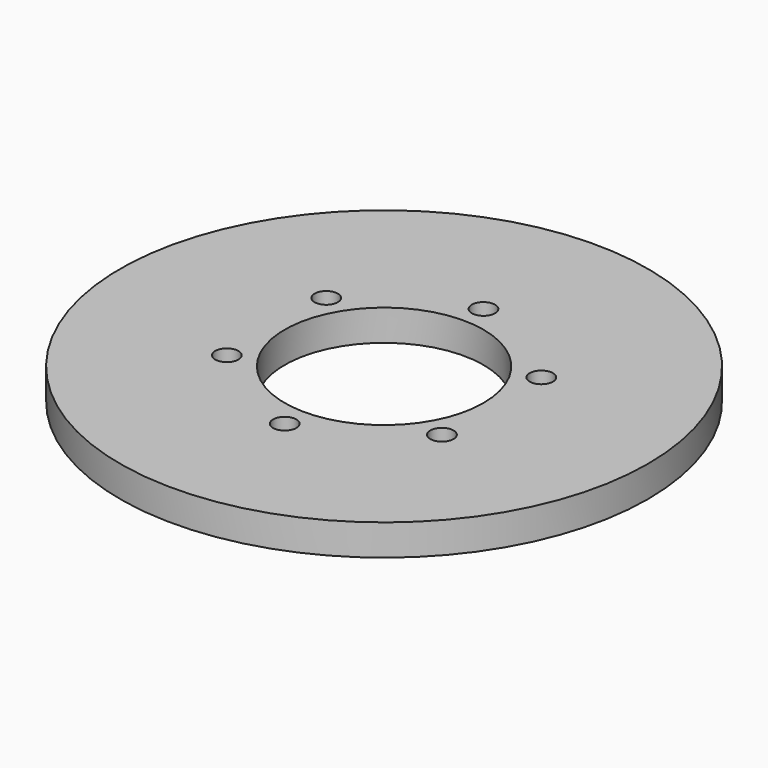
from build123d import *

# Parameters (mm, degrees)
F0_R            = 53.975
F0_R_2          = 20.32
F1_DEPTH        = 6.35
F2_D            = 4.7625
F2_DEPTH        = 6.35
F2_TIP          = 1.4307993491
F2_COPIES_COUNT = 6


# Not quite as in the source:
# - a pattern or mirror of a feature is missing from the dataset's text; its kind, count and spacing are read off the source's solid


with BuildPart() as f1:
    # F0 (on Top) → F1 (new body)
    with BuildSketch(Plane.XY):
        Circle(F0_R)
        Circle(F0_R_2, mode=Mode.SUBTRACT)
    extrude(amount=F1_DEPTH)

    # F2
    with Locations(Plane(origin=(0, 0, 0), x_dir=(1, 0, 0), z_dir=(0, 0, -1))):
        with Locations((0, 25.4)):
            f2 = Hole(F2_D / 2, depth=F2_DEPTH)
            with Locations((0, 0, -(F2_DEPTH + F2_TIP / 2))):  # 118° drill point
                Cone(0, F2_D / 2, F2_TIP, mode=Mode.SUBTRACT)

    # F2_copies: F2 ×6 about axis
    f2_copies_axis = Axis((0, 0, 0), (0, 0, 1))
    for i in range(1, F2_COPIES_COUNT):
        add(f2.rotate(f2_copies_axis, i * 360 / F2_COPIES_COUNT), mode=Mode.SUBTRACT)


solid = f1.part
